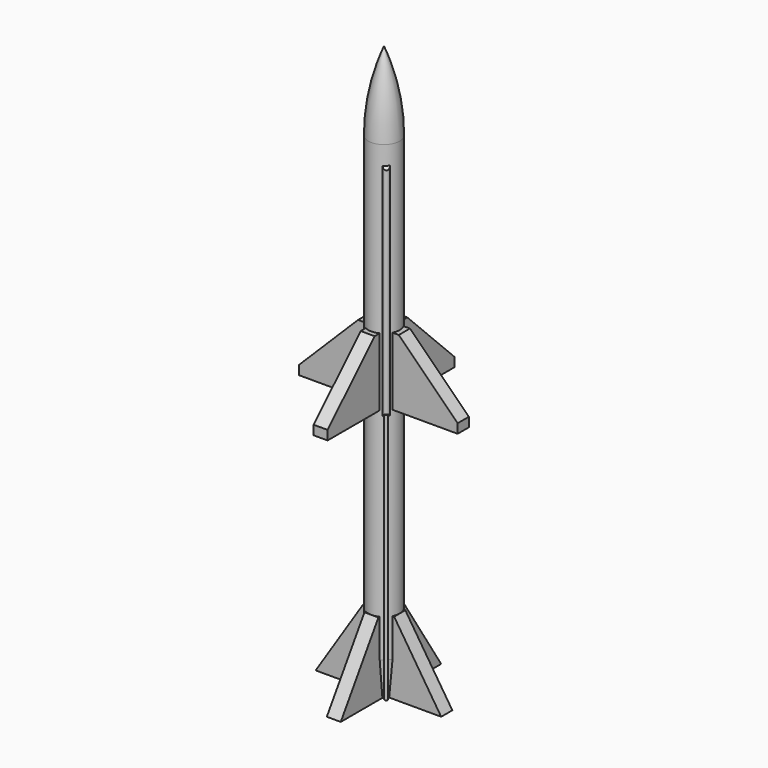
from build123d import *

# Parameters (mm, degrees)
F5_DEPTH      = 0.15
F6_COUNT      = 4
F8_DEPTH      = 4.5333333333
F10_DEPTH     = 5.5
F11_T4_ANGLE  = 108.3940583295
F11_S5_R      = 0.0625
F11_T6_DEPTH  = 2
F11_T10_ANGLE = 92.0927950404
F11_S11_R     = 0.0625
F11_T12_DEPTH = 2
F11_T16_ANGLE = 92.0927950404
F11_S17_R     = 0.0625
F11_T18_DEPTH = 2


# Not quite as in the source:
# - a fillet or chamfer that OpenCascade refuses, or shapes differently, is made with other operations: its cross-section is extruded or revolved along the edge and cut away or added


with BuildPart() as f1:
    # F0 (on Front) → F1 (revolve)
    with BuildSketch(Plane.XZ):
        with BuildLine():
            Line((0, 12.2), (0, 0))
            Line((0, 0), (0.3383333333, 0))
            Line((0.3383333333, 0), (0.3383333333, 10.51))
            ThreePointArc((0.3383333333, 10.51), (0.2529190672, 11.3717669993), (0, 12.2))
        make_face()
    revolve(axis=Axis((0, 0, 6.1), (0, 0, 1)))

    # F2 (on Front) → F3 (revolve, cut)
    with BuildSketch(Plane.XZ):
        Polygon((0.3383333333, 0.75), (0.275, 0), (0.3383333333, 0), (1.275, 0), (1.275, 0.75), align=None)
    revolve(axis=Axis((0, 0, 0), (0, 0, 1)), mode=Mode.SUBTRACT)

    # F4 (on Front) → F5 (join, symmetric)
    with BuildSketch(Plane.XZ):
        Polygon((0.3383333333, 6.9333333333), (-0.3383333333, 6.9333333333), (-0.4383333333, 6.9333333333), (-1.7039166667, 5.6733333333), (-1.7039166667, 5.4733333333), (-0.3383333333, 5.4733333333), (0.3383333333, 5.4733333333), (1.7039166667, 5.4733333333), (1.7039166667, 5.6733333333), (0.4383333333, 6.9333333333), align=None)
        Polygon((-0.06, 0.75), (-0.06, 1.5663333333), (-0.3383333333, 1.5663333333), (-1.35, 0), (-0.06, 0), align=None)
        Polygon((1.35, 0), (0.3383333333, 1.5663333333), (0.06, 1.5663333333), (0.06, 0.75), (0.06, 0), align=None)
    extrude(amount=F5_DEPTH, both=True)

    # F6: F1 ×4 about axis
    f6_axis = Axis((0, 0, 0), (0, 0, 1))


with BuildPart() as f1_1:
    add(f1.part)
    for i in range(1, F6_COUNT):
        add(f1.part.rotate(f6_axis, i * 360 / F6_COUNT))

    # F7 (on face) → F8 (join)
    with BuildSketch(Plane(origin=(0, 0, 5.4733333333), x_dir=(1, 0, 0), z_dir=(0, 0, -1))):
        with BuildLine():
            Line((0.190926215, 0.2793145626), (0.0495048587, 0.1378932064))
            Line((0.0495048587, 0.1378932064), (0.1378932064, 0.0495048587))
            Line((0.1378932064, 0.0495048587), (0.2793145626, 0.190926215))
            ThreePointArc((0.2793145626, 0.190926215), (0.2793145626, 0.2793145626), (0.190926215, 0.2793145626))
        make_face()
    extrude(amount=-F8_DEPTH)

    # F9 (on face) → F10 (join)
    with BuildSketch(Plane(origin=(0, 0, 0), x_dir=(1, 0, 0), z_dir=(0, 0, -1))):
        with BuildLine():
            ThreePointArc((0.214503642, 0.2616440941), (0.2392377943, 0.2392377943), (0.2616440941, 0.214503642))
            ThreePointArc((0.2616440941, 0.214503642), (0.2616440941, 0.2616440941), (0.214503642, 0.2616440941))
        make_face()
        with BuildLine():
            ThreePointArc((0.1694503543, 0.2165908064), (0.1944543648, 0.1944543648), (0.2165908064, 0.1694503543))
            Line((0.2165908064, 0.1694503543), (0.2616440941, 0.214503642))
            ThreePointArc((0.2616440941, 0.214503642), (0.2392377943, 0.2392377943), (0.214503642, 0.2616440941))
            Line((0.214503642, 0.2616440941), (0.1694503543, 0.2165908064))
        make_face()
    extrude(amount=-F10_DEPTH)

    # F11: chamfer of 0.1 on 3 edges, made by hand


with BuildPart() as f11_tool2:
    # F11_s3 → F11_t4 (revolve)
    with BuildSketch(Plane(origin=(0, 0, 0), x_dir=(0, 0, 1), z_dir=(-0.9871445537, 0.1598300036, 0))):
        Polygon((10.1066666667, -0.3383333333), (10.0066666667, -0.4383333333), (10.0066666667, -0.3383333333), align=None)
    revolve(axis=Axis((0, 0, 10.0066666667), (0, 0, 1)), revolution_arc=F11_T4_ANGLE)

    # F11_s5 → F11_t6 (intersect, symmetric)
    with BuildSketch(Plane.XY.offset(10.1)):
        with Locations((0.2351203888, -0.2351203888)):
            Circle(F11_S5_R)
    extrude(amount=F11_T6_DEPTH, both=True, mode=Mode.INTERSECT)


with BuildPart() as f1_2:
    add(f1_1.part)

    # F11_t1: union F11_tool2
    add(f11_tool2.part)


with BuildPart() as f11_tool8:
    # F11_s9 → F11_t10 (revolve)
    with BuildSketch(Plane(origin=(0, 0, 0), x_dir=(0, 0, 1), z_dir=(-0.9923247976, -0.123658789, 0))):
        Polygon((5.3733333333, -0.3383333333), (5.4733333333, -0.4383333333), (5.4733333333, -0.3383333333), align=None)
    revolve(axis=Axis((0, 0, 5.4733333333), (0, 0, 1)), revolution_arc=F11_T10_ANGLE)

    # F11_s11 → F11_t12 (intersect, symmetric)
    with BuildSketch(Plane.XY.offset(5.4)):
        with Locations((0.2351203888, -0.2351203888)):
            Circle(F11_S11_R)
    extrude(amount=F11_T12_DEPTH, both=True, mode=Mode.INTERSECT)


with BuildPart() as f1_3:
    add(f1_2.part)

    # F11_t7: union F11_tool8
    add(f11_tool8.part)


with BuildPart() as f11_tool14:
    # F11_s15 → F11_t16 (revolve)
    with BuildSketch(Plane(origin=(0, 0, 0), x_dir=(0, 0, 1), z_dir=(-0.9871471339, 0.1598140671, 0))):
        Polygon((5.3733333333, -0.3383333333), (5.4733333333, -0.4383333333), (5.4733333333, -0.3383333333), align=None)
    revolve(axis=Axis((0, 0, 5.4733333333), (0, 0, 1)), revolution_arc=F11_T16_ANGLE)

    # F11_s17 → F11_t18 (intersect, symmetric)
    with BuildSketch(Plane.XY.offset(5.4)):
        with Locations((0.2351203888, -0.2351203888)):
            Circle(F11_S17_R)
    extrude(amount=F11_T18_DEPTH, both=True, mode=Mode.INTERSECT)


with BuildPart() as f1_4:
    add(f1_3.part)

    # F11_t13: union F11_tool14
    add(f11_tool14.part)


solid = f1_4.part
